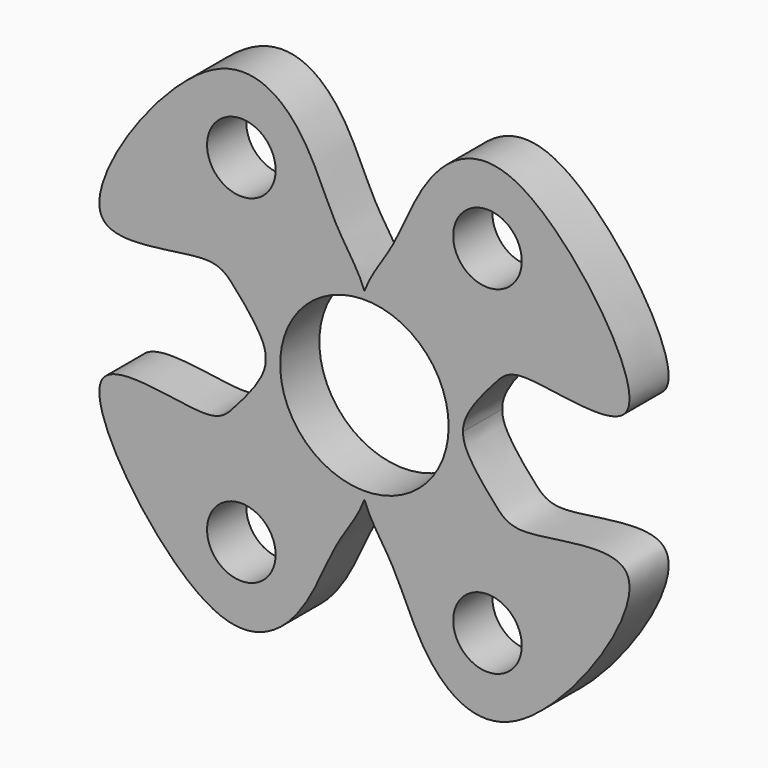
from build123d import *

# Parameters (mm, degrees)
F0_R     = 4.445
F0_R_2   = 10.922
F1_DEPTH = 6.35


# Not quite as in the source:
# - a feature of the source that left no trace in its solid (it failed there, or was rolled back) is left out


with BuildPart() as f1:
    # F0 (on Front) → F1 (new body)
    with BuildSketch(Plane.XZ):
        with BuildLine():
            add(Edge.make_bspline(
                [(0, 11.9048783648), (0.8654849169, 14.273399942), (4.2546283469, 18.1864903302), (7.7886554867, 28.8816390749), (20.4473781602, 36.3842350457), (43.2694030288, 3.1160158933), (19.7656572958, 10.2070808743), (16.889296228, 6.9029692545), (12.6311089417, 1.9755885943), (12.8090780113, 0)],
                knots=[0, 0, 0, 0, 0.1190057466, 0.2626834342, 0.4066905335, 0.6278688654, 0.7858909514, 0.8808601002, 1, 1, 1, 1], degree=3))
            add(Edge.make_bspline(
                [(0, 11.9048783648), (-0.8654849169, 14.273399942), (-4.2546283469, 18.1864903302), (-7.7886554867, 28.8816390749), (-20.4473781602, 36.3842350457), (-43.2694030288, 3.1160158933), (-19.7656572958, 10.2070808743), (-16.889296228, 6.9029692545), (-12.6311089417, 1.9755885943), (-12.8090780113, 0)],
                knots=[0, 0, 0, 0, 0.1190057466, 0.2626834342, 0.4066905335, 0.6278688654, 0.7858909514, 0.8808601002, 1, 1, 1, 1], degree=3))
            add(Edge.make_bspline(
                [(0, -11.9048783648), (-0.8654849169, -14.273399942), (-4.2546283469, -18.1864903302), (-7.7886554867, -28.8816390749), (-20.4473781602, -36.3842350457), (-43.2694030288, -3.1160158933), (-19.7656572958, -10.2070808743), (-16.889296228, -6.9029692545), (-12.6311089417, -1.9755885943), (-12.8090780113, 0)],
                knots=[0, 0, 0, 0, 0.1190057466, 0.2626834342, 0.4066905335, 0.6278688654, 0.7858909514, 0.8808601002, 1, 1, 1, 1], degree=3))
            add(Edge.make_bspline(
                [(0, -11.9048783648), (0.8654849169, -14.273399942), (4.2546283469, -18.1864903302), (7.7886554867, -28.8816390749), (20.4473781602, -36.3842350457), (43.2694030288, -3.1160158933), (19.7656572958, -10.2070808743), (16.889296228, -6.9029692545), (12.6311089417, -1.9755885943), (12.8090780113, 0)],
                knots=[0, 0, 0, 0, 0.1190057466, 0.2626834342, 0.4066905335, 0.6278688654, 0.7858909514, 0.8808601002, 1, 1, 1, 1], degree=3))
        make_face()
        with Locations((-15.9579783894, -21.950429026)):
            Circle(F0_R, mode=Mode.SUBTRACT)
        with Locations((15.9579783894, -21.950429026)):
            Circle(F0_R, mode=Mode.SUBTRACT)
        with Locations((-15.9579783894, 21.950429026)):
            Circle(F0_R, mode=Mode.SUBTRACT)
        Circle(F0_R_2, mode=Mode.SUBTRACT)
        with Locations((15.9579783894, 21.950429026)):
            Circle(F0_R, mode=Mode.SUBTRACT)
    extrude(amount=F1_DEPTH)


solid = f1.part
